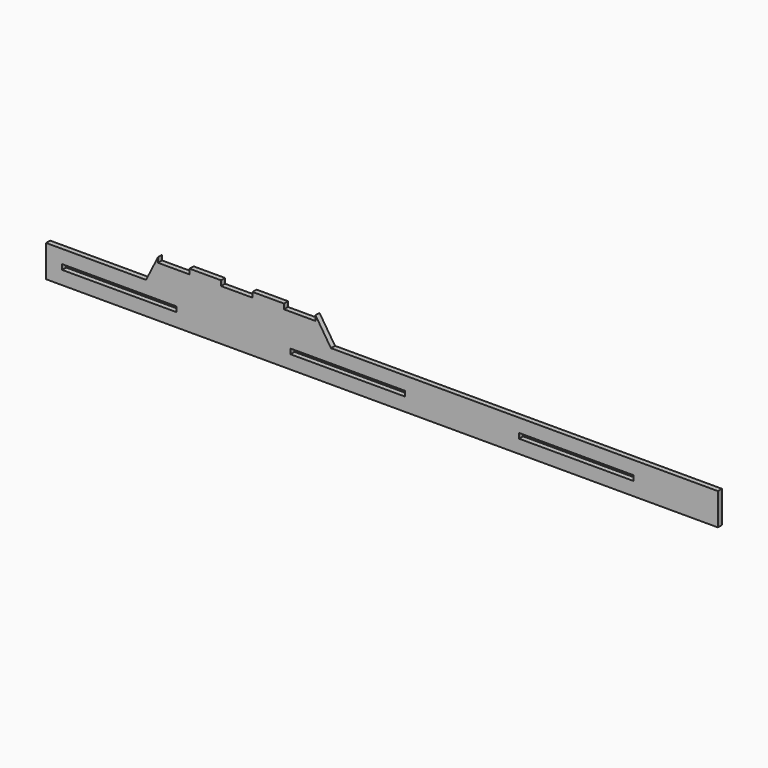
from build123d import *

# Parameters (mm, degrees)
F0_W     = 71.4285714286
F0_H     = 3.175
F1_DEPTH = 3.175


# Not quite as in the source:
# - ends of sketch curves that miss each other by under 0.0002 mm in the source are joined


with BuildPart() as f1:
    # F0 (on Front) → F1 (new body)
    with BuildSketch(Plane.XZ):
        Polygon((-260, 10), (-260, -10), (160, -10), (160, 10), (-81.8902254105, 10), (-91.575, 10), (-190, 10), (-197.4899102798, 10), align=None)
        with Locations((-214.2857571429, 0)):
            Rectangle(F0_W, F0_H, mode=Mode.SUBTRACT)
        Polygon((-35.7142857143, 1.5875), (-35.7142857143, -1.5875), (-107.1428714286, -1.5875), (-107.1428857143, 1.5875), align=None, mode=Mode.SUBTRACT)
        with Locations((71.4285857143, 0)):
            Rectangle(F0_W, F0_H, mode=Mode.SUBTRACT)
        Polygon((-190, 25), (-197.4899102798, 10), (-190, 10), (-190, 21.825), align=None)
        Polygon((-190, 21.825), (-190, 10), (-91.575, 10), (-91.575, 21.825), (-111.26, 21.825), (-111.26, 25), (-130.945, 25), (-130.945, 21.825), (-150.63, 21.825), (-150.63, 25), (-170.315, 25), (-170.315, 21.825), align=None)
        Polygon((-91.575, 10), (-81.8902254105, 10), (-91.575, 25), (-91.575, 21.825), align=None)
    extrude(amount=F1_DEPTH)


solid = f1.part
